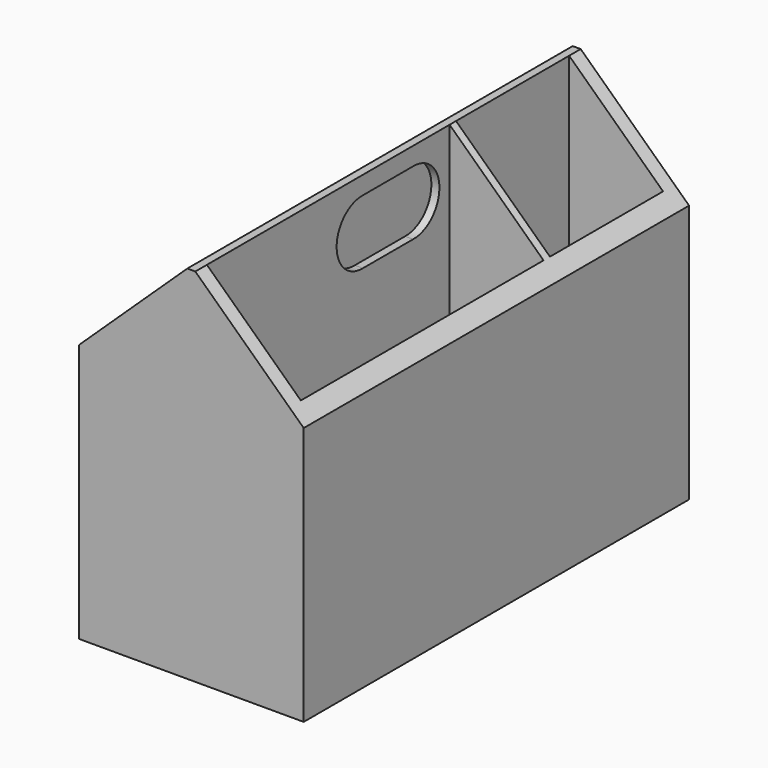
from build123d import *

# Parameters (mm, degrees)
F0_W     = 88.9
F0_H     = 190.5
F0_W_2   = 82.55
F0_H_2   = 184.15
F1_DEPTH = 3.175
F2_W     = 88.9
F2_H     = 190.5
F2_W_2   = 3.175
F2_H_2   = 3.175
F2_W_3   = 37.1475
F2_H_3   = 58.1914
F2_H_4   = 55.9145467066
F2_H_5   = 58.6140532934
F3_DEPTH = 139.7
F6_DEPTH = 190.5
F8_DEPTH = 25.4


# Not quite as in the source:
# - a feature names something its author has since deleted; it is built from what else it names


with BuildPart() as f1:
    # F0 (on Top) → F1 (new body)
    with BuildSketch(Plane.XY):
        Rectangle(F0_W, F0_H)
        Rectangle(F0_W_2, F0_H_2, mode=Mode.SUBTRACT)
        Rectangle(F0_W_2, F0_H_2)
    extrude(amount=F1_DEPTH)

    # F2 (on face) → F3 (join)
    with BuildSketch(Plane.XY.offset(3.175)):
        Rectangle(F2_W, F2_H)
        Polygon((-1.5875, -89.535), (-38.735, -89.535), (-38.735, -30.9209467066), (-38.735, -27.7459467066), (-38.735, 89.535), (-1.5875, 89.535), (1.5875, 89.535), (38.735, 89.535), (38.735, 33.6204532934), (38.735, 30.4454532934), (38.735, -89.535), (1.5875, -89.535), align=None, mode=Mode.SUBTRACT)
        with Locations((0, 32.0329532934)):
            Rectangle(F2_W_2, F2_H_2)
        with Locations((20.16125, 32.0329532934)):
            Rectangle(F2_W_3, F2_H_2)
        with Locations((-20.16125, -29.3334467066)):
            Rectangle(F2_W_3, F2_H_2)
        with Locations((0, -29.3334467066)):
            Rectangle(F2_W_2, F2_H_2)
        with Locations((0, 1.3497532934)):
            Rectangle(F2_W_2, F2_H_3)
        with Locations((0, 61.5777266467)):
            Rectangle(F2_W_2, F2_H_4)
        with Locations((0, -60.2279733533)):
            Rectangle(F2_W_2, F2_H_5)
    extrude(amount=F3_DEPTH)

    # F5 (on face) → F6 (cut)
    with BuildSketch(Plane.XZ.offset(95.25)):
        Polygon((-44.45, 102.3109257221), (-1.5860880958, 142.875), (-44.45, 142.875), align=None)
        Polygon((44.45, 142.875), (1.5860880958, 142.875), (44.45, 102.3109257221), align=None)
    extrude(amount=-F6_DEPTH, mode=Mode.SUBTRACT)

    # F7 (on face) → F8 (cut)
    with BuildSketch(Plane.YZ.offset(1.5875)):
        with BuildLine():
            Line((12.7, 135.732749784), (0, 135.732749784))
            Line((0, 135.732749784), (-12.7, 135.732749784))
            ThreePointArc((-12.7, 135.732749784), (-25.4008333473, 122.8855821986), (-12.4090174213, 110.332749784))
            Line((-12.4090174213, 110.332749784), (0, 110.332749784))
            Line((0, 110.332749784), (12.4090174213, 110.332749784))
            ThreePointArc((12.4090174213, 110.332749784), (25.4008333473, 122.8855821986), (12.7, 135.732749784))
        make_face()
    extrude(amount=-F8_DEPTH, mode=Mode.SUBTRACT)


solid = f1.part
